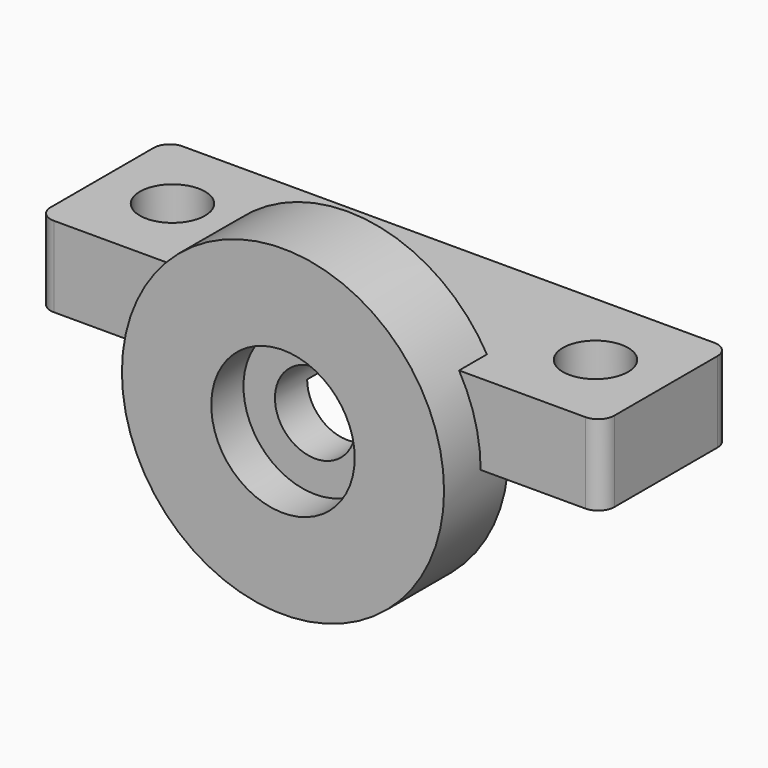
from build123d import *

# Parameters (mm, degrees)
F0_R      = 50.8
F0_R_2    = 12.7
F1_DEPTH  = 25.4
F2_W      = 177.8
F2_H      = 50.8
F3_DEPTH  = 25.4
F5_R      = 22.6237609961
F6_DEPTH  = 12.7
F7_R      = 10.2865280917
F8_DEPTH  = 25.4
F9_R      = 5.08
F11_R     = 12.7
F12_DEPTH = 76.2


# Not quite as in the source:
# - a feature names something its author has since deleted; it is built from what else it names


with BuildPart() as f1:
    # F0 (on Front) → F1 (new body)
    with BuildSketch(Plane.XZ):
        Circle(F0_R)
        Circle(F0_R_2, mode=Mode.SUBTRACT)
    extrude(amount=F1_DEPTH)

    # F2 (on Top) → F3 (join)
    with BuildSketch(Plane.XY):
        with Locations((0, 14.4235261992)):
            Rectangle(F2_W, F2_H)
    extrude(amount=F3_DEPTH)

    # F4: union 

    # F5 (on face) → F6 (cut)
    with BuildSketch(Plane.XZ.offset(25.4)):
        Circle(F5_R)
    extrude(amount=-F6_DEPTH, mode=Mode.SUBTRACT)

    # F7 (on face) → F8 (cut)
    with BuildSketch(Plane.XY.offset(25.4)):
        with Locations((-66.7031380003, 14.4235261992)):
            Circle(F7_R)
        with Locations((66.7031380003, 14.4235261992)):
            Circle(F7_R)
    extrude(amount=-F8_DEPTH, mode=Mode.SUBTRACT)

    # F9
    f9_edges = [f1.edges().sort_by_distance(p)[0] for p in [
        (88.9, 39.823526, 12.7),
        (-88.9, 39.823526, 12.7),
        (-88.9, -10.976474, 12.7),
        (88.9, -10.976474, 12.7),
    ]]
    fillet(f9_edges, radius=F9_R)

    # F11 (on face) → F12 (cut)
    with BuildSketch(Plane.XZ.offset(25.4)):
        Circle(F11_R)
    extrude(amount=-F12_DEPTH, mode=Mode.SUBTRACT)


solid = f1.part
